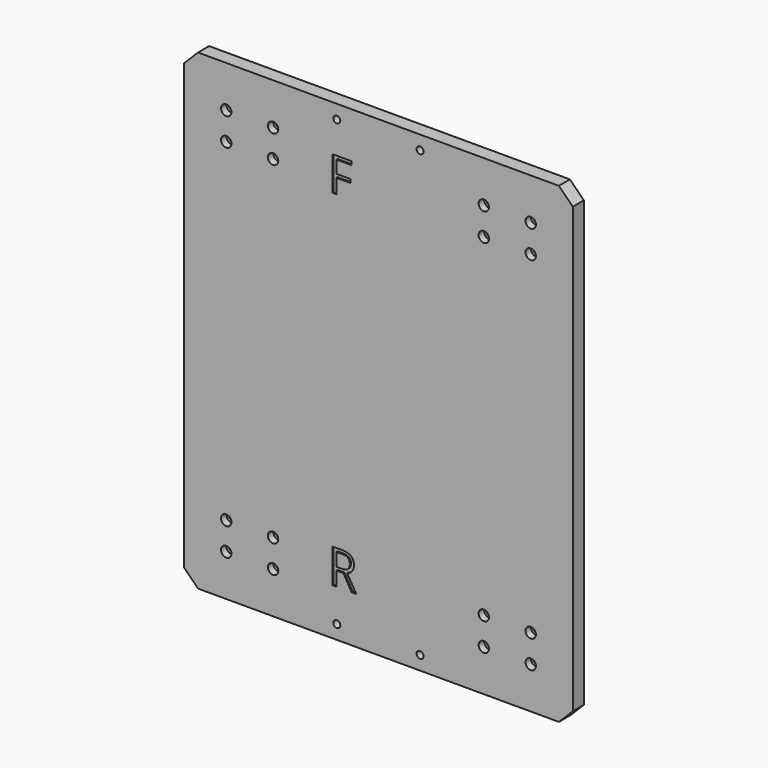
from build123d import *

# Parameters (mm, degrees)
F0_W           = 355.6
F0_H           = 431.8
F1_DEPTH       = 12.7
F2_SIZE2       = 12.7
F2_SIZE        = 12.7
F4_D           = 4.7625
F4_CBORE_D     = 9.525
F4_CBORE_DEPTH = 6.35
F6_D           = 6.35
F6_DEPTH       = 9.525
F6_TIP         = 1.9077324654
F7_TEXT_SIZE   = 43.7091666667
F8_DEPTH       = 1.27


# Not quite as in the source:
# - Text() gives the source's letters only with a copy of the font that has no kerning and outlines rounded to 1/6400 em; it was checked with that copy


with BuildPart() as f1:
    # F0 (on Front) → F1 (new body)
    with BuildSketch(Plane.XZ):
        with Locations((-46.1366650008, 13.7544050813)):
            Rectangle(F0_W, F0_H)
    extrude(amount=F1_DEPTH)

    # F2
    f2_edges = [f1.edges().sort_by_distance(p)[0] for p in [
        (-223.936665, -6.35, 229.654405),
        (131.663335, -6.35, 229.654405),
        (131.663335, -6.35, -202.145595),
        (-223.936665, -6.35, -202.145595),
    ]]
    chamfer(f2_edges, length=F2_SIZE, length2=F2_SIZE2)

    # F4 (through all)
    with Locations(Plane.XZ.offset(12.7)):
        with Locations((-185.4302650008, 166.1544050813), (-142.5550650008, 166.1544050813), (-142.5550650008, 191.5544050813), (-185.4302650008, 191.5544050813), (50.2817349992, 166.1544050813), (-185.4302650008, -164.0455949187), (-185.4302650008, -138.6455949187), (93.1569349992, 166.1544050813), (93.1569349992, 191.5544050813), (-142.5550650008, -164.0455949187), (50.2817349992, -138.6455949187), (50.2817349992, 191.5544050813), (-142.5550650008, -138.6455949187), (93.1569349992, -138.6455949187), (93.1569349992, -164.0455949187), (50.2817349992, -164.0455949187)):
            CounterBoreHole(F4_D / 2, F4_CBORE_D / 2, F4_CBORE_DEPTH)

    # F6
    with Locations(Plane.XZ.offset(12.7)):
        with Locations((-84.2366650008, 216.9544050813), (-8.0366650008, 216.9544050813), (-8.0366650008, -189.4455949187), (-84.2366650008, -189.4455949187)):
            Hole(F6_D / 2, depth=F6_DEPTH)
            with Locations((0, 0, -(F6_DEPTH + F6_TIP / 2))):  # 118° drill point
                Cone(0, F6_D / 2, F6_TIP, mode=Mode.SUBTRACT)

    # F7 (on face) → F8 (cut)
    with BuildSketch(Plane.XZ.offset(12.7)):
        with Locations((-92.6186650008, 156.5819046852)):
            Text('F', F7_TEXT_SIZE, font='Open Sans', text_align=(TextAlign.LEFT, TextAlign.BOTTOM))
        with Locations((-92.6186650008, -159.4213236839)):
            Text('R', F7_TEXT_SIZE, font='Open Sans', text_align=(TextAlign.LEFT, TextAlign.BOTTOM))
    extrude(amount=-F8_DEPTH, mode=Mode.SUBTRACT)


solid = f1.part
